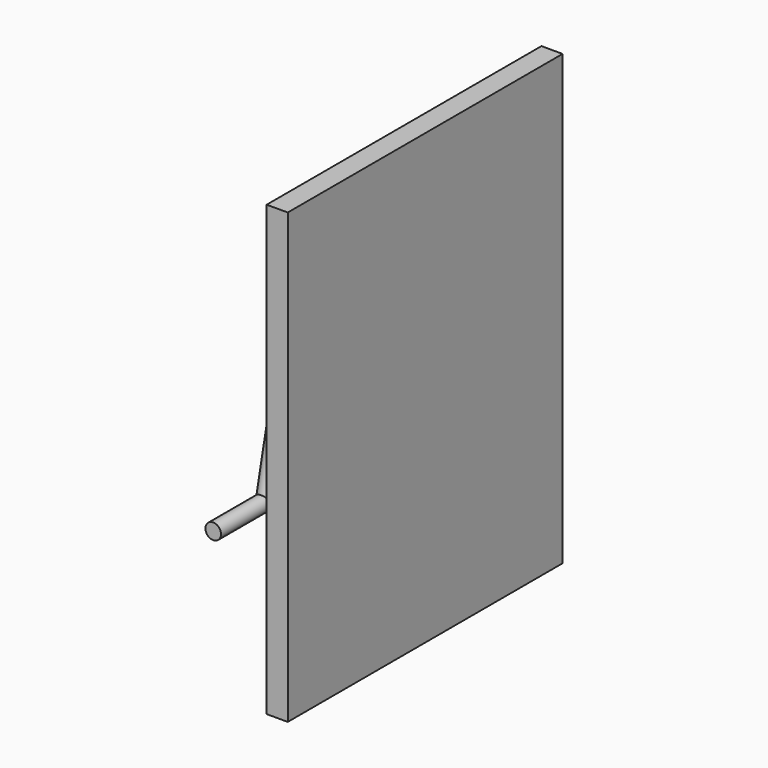
from build123d import *

# Parameters (mm, degrees)
F0_R          = 13.3086591282
F3_W          = 36.0237117857
F3_H          = 585.9275087714
F4_DEPTH      = 500
F4_DEPTH_BACK = 95
F5_R          = 9.0158495844
F6_DEPTH      = 80
F5_R_2        = 8.5543973975
F5_R_3        = 8.9567769952
F5_R_4        = 8.5868004183
F8_W          = 62.6919232309
F8_H          = 24.4294032454
F9_DEPTH      = 30.8
F12_DEPTH     = 90.5
F13_W         = 16.1430759363
F13_H         = 18.8865625858
F14_DEPTH     = 404
F15_DEPTH     = 265
F16_R         = 8.3021782339
F17_DEPTH     = 50
F16_R_2       = 7.0466149253
F19_T1_DEPTH  = 16.1430759363
F19_T3_DEPTH  = 41.1430759363
F19_T6_ANGLE  = 168.7003231043


# Not quite as in the source:
# - a fillet or chamfer that OpenCascade refuses, or shapes differently, is made with other operations: its cross-section is extruded or revolved along the edge and cut away or added


with BuildPart() as f2:
    # F2: sweep along a path in F1
    with BuildLine(Plane.YZ) as f2_path:
        Line((0, 64.4181072712), (-13.9453124047, 64.4181072712))
        Line((-13.9453124047, 64.4181072712), (-73.1850613519, -202.2097110748))
        Line((-73.1850613519, -202.2097110748), (-185.0498318672, -202.2097110748))
    # F0 (on Front) → F2 (sweep)
    with BuildSketch(Plane.XZ):
        with Locations((0, 64.417861402)):
            Circle(F0_R)
    sweep(path=f2_path.line, transition=Transition.RIGHT)


with BuildPart() as f4:
    # F3 (on Top) → F4 (new body, two sides)
    with BuildSketch(Plane.XY) as f4_sk:
        with Locations((45.6317188218, 187.2877962887)):
            Rectangle(F3_W, F3_H)
    extrude(amount=-F4_DEPTH)
    extrude(f4_sk.sketch, amount=F4_DEPTH_BACK)

    # F3 (on Top) → F15 (join)
    with BuildSketch(Plane.XY):
        with Locations((45.6317188218, 187.2877962887)):
            Rectangle(F3_W, F3_H)
    extrude(amount=F15_DEPTH)


with BuildPart() as f6:
    # F5 (on face) → F6 (new body)
    with BuildSketch(Plane(origin=(27.619862929, 0, 0), x_dir=(0, -1, 0), z_dir=(-1, 0, 0))):
        with Locations((73.3310803771, -202.0987272263)):
            Circle(F5_R)
    extrude(amount=F6_DEPTH)


with BuildPart() as f6b:
    # F5 (on face) → F6, piece 2 (new body)
    with BuildSketch(Plane(origin=(27.619862929, 0, 0), x_dir=(0, -1, 0), z_dir=(-1, 0, 0))):
        with Locations((14.3033554778, 64.6395683289)):
            Circle(F5_R_2)
    extrude(amount=F6_DEPTH)


with BuildPart() as f6c:
    # F5 (on face) → F6, piece 3 (new body)
    with BuildSketch(Plane(origin=(27.619862929, 0, 0), x_dir=(0, -1, 0), z_dir=(-1, 0, 0))):
        with Locations((56.9279193878, -132.585093379)):
            Circle(F5_R_3)
    extrude(amount=F6_DEPTH)


with BuildPart() as f6d:
    # F5 (on face) → F6, piece 4 (new body)
    with BuildSketch(Plane(origin=(27.619862929, 0, 0), x_dir=(0, -1, 0), z_dir=(-1, 0, 0))):
        with Locations((29.2789824307, 0)):
            Circle(F5_R_4)
    extrude(amount=F6_DEPTH)


with BuildPart() as f2_1:
    add(f2.part)

    # F7: cut F6d, F6c, F6, F6b
    add(f6d.part, mode=Mode.SUBTRACT)
    add(f6c.part, mode=Mode.SUBTRACT)
    add(f6.part, mode=Mode.SUBTRACT)
    add(f6b.part, mode=Mode.SUBTRACT)


with BuildPart() as f9:
    # F8 (on Front) → F9 (new body)
    with BuildSketch(Plane.XZ):
        with Locations((4.9693156034, 87.2141830623)):
            Rectangle(F8_W, F8_H)
    extrude(amount=F9_DEPTH)


with BuildPart() as f2_2:
    add(f2_1.part)

    # F10: cut F9
    add(f9.part, mode=Mode.SUBTRACT)

    # F11 (on face) → F12 (join)
    with BuildSketch(Plane.XY.offset(74.9994814396)):
        with BuildLine():
            Line((8.0715379682, -22.4337283609), (8.0715379682, -0.7198430731))
            ThreePointArc((8.0715379682, -0.7198430731), (7.5435055203, -0.3471123394), (6.9982904346, 0))
            Line((6.9982904346, 0), (-6.9982904346, 0))
            ThreePointArc((-6.9982904346, 0), (-7.5435055203, -0.3471123394), (-8.0715379682, -0.7198430731))
            Line((-8.0715379682, -0.7198430731), (-8.0715379682, -22.4337283609))
            Line((-8.0715379682, -22.4337283609), (8.0715379682, -22.4337283609))
        make_face()
        with BuildLine():
            ThreePointArc((-7.0667591259, -23.1465463218), (0, -25.1365519195), (7.0667591259, -23.1465463218))
            add(Edge.make_bspline(
                [(7.0667591259, -23.1465463218), (7.5851413227, -22.8137933841), (8.0715379682, -22.4337283609)],
                knots=[6.8375555203, 6.8375555203, 6.8375555203, 6.9348209354, 6.9348209354, 6.9348209354], degree=2, weights=[0.9716974687, 0.9847074225, 1]))
            Line((8.0715379682, -22.4337283609), (-8.0715379682, -22.4337283609))
            add(Edge.make_bspline(
                [(-8.0715379682, -22.4337283609), (-7.5851413227, -22.8137933841), (-7.0667591259, -23.1465463218)],
                knots=[5.631549679, 5.631549679, 5.631549679, 5.7288150941, 5.7288150941, 5.7288150941], degree=2, weights=[1, 0.9847074225, 0.9716974687]))
        make_face()
        with BuildLine():
            ThreePointArc((6.9982904346, 0), (7.5435055203, -0.3471123394), (8.0715379682, -0.7198430731))
            Line((8.0715379682, -0.7198430731), (8.0715379682, 0))
            Line((8.0715379682, 0), (6.9982904346, 0))
        make_face()
        with BuildLine():
            ThreePointArc((-8.0715379682, -0.7198430731), (-7.5435055203, -0.3471123394), (-6.9982904346, 0))
            Line((-6.9982904346, 0), (-8.0715379682, 0))
            Line((-8.0715379682, 0), (-8.0715379682, -0.7198430731))
        make_face()
    extrude(amount=F12_DEPTH)

    # F13 (on face) → F14 (join)
    with BuildSketch(Plane(origin=(0, 0, 0), x_dir=(-1, 0, 0), z_dir=(0, 1, 0))):
        with Locations((0, 156.0562001467)):
            Rectangle(F13_W, F13_H)
    extrude(amount=F14_DEPTH)


with BuildPart() as f17:
    # F16 (on face) → F17 (new body)
    with BuildSketch(Plane(origin=(27.619862929, 0, 0), x_dir=(0, -1, 0), z_dir=(-1, 0, 0))):
        with Locations((11.4515069872, 155.9651345015)):
            Circle(F16_R)
    extrude(amount=F17_DEPTH)


with BuildPart() as f17b:
    # F16 (on face) → F17, piece 2 (new body)
    with BuildSketch(Plane(origin=(27.619862929, 0, 0), x_dir=(0, -1, 0), z_dir=(-1, 0, 0))):
        with Locations((-397.8760838509, 155.8553129435)):
            Circle(F16_R_2)
    extrude(amount=F17_DEPTH)


with BuildPart() as f2_3:
    add(f2_2.part)

    # F18: cut F17b, F17
    add(f17b.part, mode=Mode.SUBTRACT)
    add(f17.part, mode=Mode.SUBTRACT)

    # F19: fillet of radius 5 on 4 edges, made by hand

    # F19_s2 → F19_t1 (join)
    with BuildSketch(Plane.YZ.offset(-8.0715379682)):
        with BuildLine():
            ThreePointArc((5, 146.6129188538), (1.4644660941, 145.1484527597), (0, 141.6129188538))
            Line((0, 141.6129188538), (0, 146.6129188538))
            Line((0, 146.6129188538), (5, 146.6129188538))
        make_face()
    extrude(amount=F19_T1_DEPTH)

    # F19_s4 → F19_t3 (cut)
    with BuildSketch(Plane.YZ.offset(-20.5715379682)):
        with BuildLine():
            ThreePointArc((404, 160.4994814396), (402.5355339059, 164.0350153455), (399, 165.4994814396))
            Line((399, 165.4994814396), (404, 165.4994814396))
            Line((404, 165.4994814396), (404, 160.4994814396))
        make_face()
        with BuildLine():
            ThreePointArc((399, 146.6129188538), (402.5355339059, 148.0773849478), (404, 151.6129188538))
            Line((404, 151.6129188538), (404, 146.6129188538))
            Line((404, 146.6129188538), (399, 146.6129188538))
        make_face()
    extrude(amount=F19_T3_DEPTH, mode=Mode.SUBTRACT)

    # F19_s5 → F19_t6 (revolve, cut)
    with BuildSketch(Plane(origin=(1.1358751611, -11.4817045831, 0), x_dir=(0, 0, 1), z_dir=(-0.0984485563, 0.9951421415, 0))):
        with BuildLine():
            ThreePointArc((165.4994814396, -9.6838962015), (164.0350153455, -13.2194301075), (160.4994814396, -14.6838962015))
            Line((160.4994814396, -14.6838962015), (165.4994814396, -14.6838962015))
            Line((165.4994814396, -14.6838962015), (165.4994814396, -9.6838962015))
        make_face()
    revolve(axis=Axis((0, -11.594075736, 165.4994814396), (0, 0, 1)), revolution_arc=F19_T6_ANGLE, mode=Mode.SUBTRACT)


solid = Compound([f4.part, f2_3.part])
